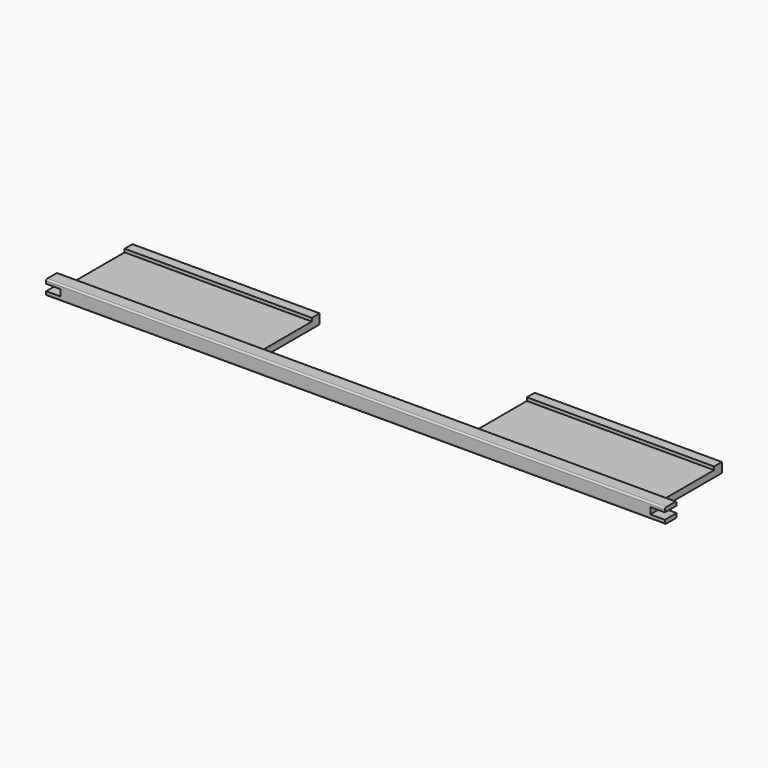
from build123d import *

# Parameters (mm, degrees)
F0_W      = 45
F0_H      = 45
F1_DEPTH  = 950
F2_R      = 5
F3_W      = 45
F3_H      = 20
F4_DEPTH  = 45.001
F5_W      = 40
F5_H      = 20
F6_DEPTH  = 25
F7_W      = 40
F7_H      = 20
F8_DEPTH  = 25
F9_W      = 575
F9_H      = 20
F10_DEPTH = 230
F11_W     = 575
F11_H     = 30
F12_DEPTH = 10


# Not quite as in the source:
# - a pattern or mirror of a feature is missing from the dataset's text; its kind, count and spacing are read off the source's solid


with BuildPart() as f1:
    # F0 (on Right) → F1 (new body, symmetric)
    with BuildSketch(Plane.YZ):
        with Locations((22.5, 22.5)):
            Rectangle(F0_W, F0_H)
    extrude(amount=F1_DEPTH, both=True)

    # F2
    f2_edges = [f1.edges().sort_by_distance(p)[0] for p in [
        (0, 0, 45),
        (0, 45, 45),
        (0, 0, 0),
        (0, 45, 0),
    ]]
    fillet(f2_edges, radius=F2_R)

    # F3 (on face) → F4 (cut, through all)
    with BuildSketch(Plane.XZ):
        with Locations((-927.5, 22.5)):
            Rectangle(F3_W, F3_H)
    f4 = extrude(amount=-F4_DEPTH, mode=Mode.SUBTRACT)

    # F4_copies: F4 across plane
    add(f4.mirror(Plane(origin=(0, 0, 0), x_dir=(0, 0, 1), z_dir=(1, 0, 0))), mode=Mode.SUBTRACT)

    # F5 (on face) → F6 (cut)
    with BuildSketch(Plane(origin=(0, 0, 0), x_dir=(1, 0, 0), z_dir=(0, 0, -1))):
        with Locations((-780, -22.5)):
            Rectangle(F5_W, F5_H)
    f6 = extrude(amount=-F6_DEPTH, mode=Mode.SUBTRACT)

    # F6_copies: F6 across plane
    add(f6.mirror(Plane(origin=(0, 0, 0), x_dir=(0, 0, 1), z_dir=(1, 0, 0))), mode=Mode.SUBTRACT)

    # F7 (on face) → F8 (cut)
    with BuildSketch(Plane(origin=(0, 0, 0), x_dir=(1, 0, 0), z_dir=(0, 0, -1))):
        with Locations((0, -22.5)):
            Rectangle(F7_W, F7_H)
    extrude(amount=-F8_DEPTH, mode=Mode.SUBTRACT)

    # F9 (on face) → F10 (join)
    with BuildSketch(Plane(origin=(0, 45, 0), x_dir=(-1, 0, 0), z_dir=(0, 1, 0))):
        with Locations((-617.5, 22.5)):
            Rectangle(F9_W, F9_H)
        with Locations((617.5, 22.5)):
            Rectangle(F9_W, F9_H)
    extrude(amount=F10_DEPTH)

    # F11 (on face) → F12 (join)
    with BuildSketch(Plane.XY.offset(32.5)):
        with Locations((-617.5, 260)):
            Rectangle(F11_W, F11_H)
        with Locations((617.5, 260)):
            Rectangle(F11_W, F11_H)
    extrude(amount=F12_DEPTH)


solid = f1.part
